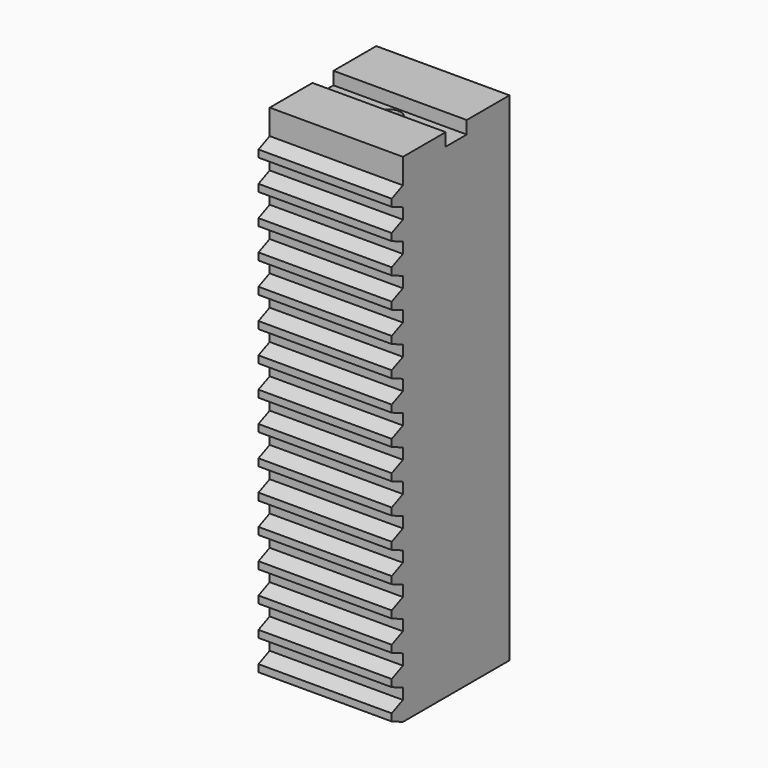
from build123d import *

# Parameters (mm, degrees)
F1_DEPTH = 9.525
F3_DEPTH = 34.6458181739


# Not quite as in the source:
# - a feature names something its author has since deleted; it is built from what else it names


with BuildPart() as f1:
    # F0 (on Right) → F1 (new body)
    with BuildSketch(Plane.YZ):
        Polygon((0, 1.3819878222), (0, 0), (9.525, 0), (9.525, 35.56), (5.7011166342, 35.56), (5.7011166342, 34.6458181739), (4.7625, 34.6458181739), (3.8238833658, 34.6458181739), (3.8238833658, 35.56), (0, 35.56), (0, 33.7669878222), (0, 32.385), (0, 31.6079878222), (0, 30.226), (0, 29.4489878222), (0, 28.067), (0, 27.2899878222), (0, 25.908), (0, 25.1309878222), (0, 23.749), (0, 22.9719878222), (0, 21.59), (0, 20.8129878222), (0, 19.431), (0, 18.6539878222), (0, 17.272), (0, 16.4949878222), (0, 15.113), (0, 14.3359878222), (0, 12.954), (0, 12.1769878222), (0, 10.795), (0, 10.0179878222), (0, 8.636), (0, 7.8589878222), (0, 6.477), (0, 5.6999878222), (0, 4.318), (0, 3.5409878222), (0, 2.159), align=None)
        Polygon((-1.00000054, 0.4354505218), (0, 0), (0, 1.3819878222), (-1.00000054, 0.9465373005), (-1.00000054, 0.6909939111), align=None)
        Polygon((-1.00000054, 2.5944505218), (0, 2.159), (0, 3.5409878222), (-1.00000054, 3.1055373005), (-1.00000054, 2.8499939111), align=None)
        Polygon((-1.00000054, 4.7534505218), (0, 4.318), (0, 5.6999878222), (-1.00000054, 5.2645373005), (-1.00000054, 5.0089939111), align=None)
        Polygon((-1.00000054, 6.9124505218), (0, 6.477), (0, 7.8589878222), (-1.00000054, 7.4235373005), (-1.00000054, 7.1679939111), align=None)
        Polygon((-1.00000054, 9.0714505218), (0, 8.636), (0, 10.0179878222), (-1.00000054, 9.5825373005), (-1.00000054, 9.3269939111), align=None)
        Polygon((-1.00000054, 11.2304505218), (0, 10.795), (0, 12.1769878222), (-1.00000054, 11.7415373005), (-1.00000054, 11.4859939111), align=None)
        Polygon((-1.00000054, 13.3894505218), (0, 12.954), (0, 14.3359878222), (-1.00000054, 13.9005373005), (-1.00000054, 13.6449939111), align=None)
        Polygon((-1.00000054, 15.5484505218), (0, 15.113), (0, 16.4949878222), (-1.00000054, 16.0595373005), (-1.00000054, 15.8039939111), align=None)
        Polygon((-1.00000054, 17.7074505218), (0, 17.272), (0, 18.6539878222), (-1.00000054, 18.2185373005), (-1.00000054, 17.9629939111), align=None)
        Polygon((-1.00000054, 19.8664505218), (0, 19.431), (0, 20.8129878222), (-1.00000054, 20.3775373005), (-1.00000054, 20.1219939111), align=None)
        Polygon((0, 21.59), (0, 22.9719878222), (-1.00000054, 22.5365373005), (-1.00000054, 22.2809939111), (-1.00000054, 22.0254505218), align=None)
        Polygon((0, 23.749), (0, 25.1309878222), (-1.00000054, 24.6955373005), (-1.00000054, 24.4399939111), (-1.00000054, 24.1844505218), align=None)
        Polygon((0, 25.908), (0, 27.2899878222), (-1.00000054, 26.8545373005), (-1.00000054, 26.5989939111), (-1.00000054, 26.3434505218), align=None)
        Polygon((0, 28.067), (0, 29.4489878222), (-1.00000054, 29.0135373005), (-1.00000054, 28.7579939111), (-1.00000054, 28.5024505218), align=None)
        Polygon((0, 30.226), (0, 31.6079878222), (-1.00000054, 31.1725373005), (-1.00000054, 30.9169939111), (-1.00000054, 30.6614505218), align=None)
        Polygon((0, 32.385), (0, 33.7669878222), (-1.00000054, 33.3315373005), (-1.00000054, 33.0759939111), (-1.00000054, 32.8204505218), align=None)
    extrude(amount=F1_DEPTH)

    # F2 (on face) → F3 (cut, through all)
    with BuildSketch(Plane.XY.offset(34.6458181739)):
        with BuildLine():
            Line((4.7625, 3.96875), (4.7625, 4.7625))
            Line((4.7625, 4.7625), (3.96875, 4.7625))
            ThreePointArc((3.96875, 4.7625), (4.2012339924, 4.2012339924), (4.7625, 3.96875))
        make_face()
        with BuildLine():
            Line((3.96875, 4.7625), (4.7625, 4.7625))
            Line((4.7625, 4.7625), (4.7625, 5.55625))
            ThreePointArc((4.7625, 5.55625), (4.2012339924, 5.3237660076), (3.96875, 4.7625))
        make_face()
        with BuildLine():
            ThreePointArc((4.7625, 3.96875), (5.3237660076, 4.2012339924), (5.55625, 4.7625))
            Line((5.55625, 4.7625), (4.7625, 4.7625))
            Line((4.7625, 4.7625), (4.7625, 3.96875))
        make_face()
        with BuildLine():
            Line((4.7625, 4.7625), (5.55625, 4.7625))
            ThreePointArc((5.55625, 4.7625), (5.3237660076, 5.3237660076), (4.7625, 5.55625))
            Line((4.7625, 5.55625), (4.7625, 4.7625))
        make_face()
    extrude(amount=-F3_DEPTH, mode=Mode.SUBTRACT)


solid = f1.part
